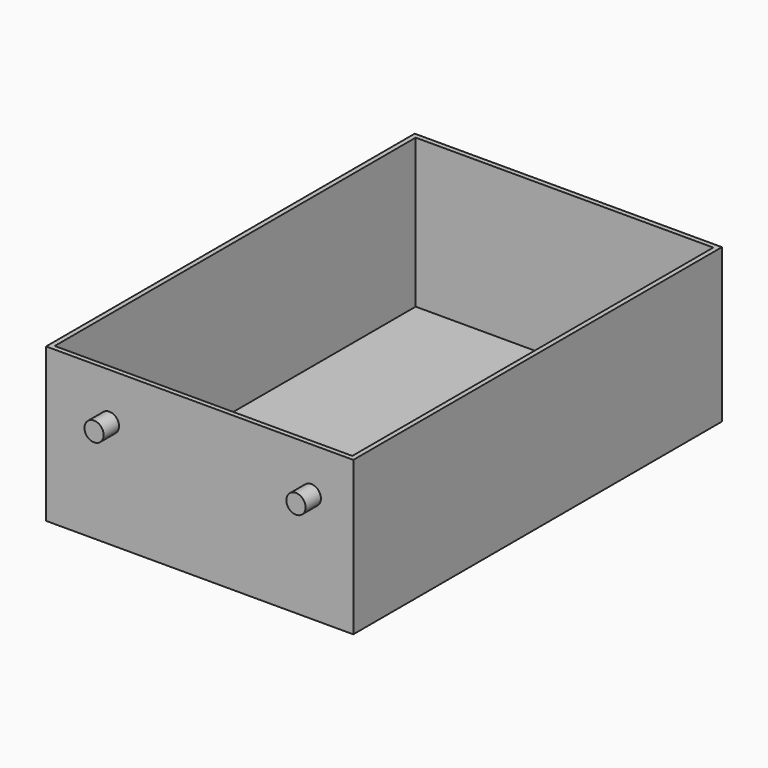
from build123d import *

# Parameters (mm, degrees)
F1_W      = 160
F1_H      = 80
F2_DEPTH  = 120
F5_T      = -2.5
F7_R      = 5
F9_DEPTH  = 10
F11_R     = 5
F12_DEPTH = 10


# Not quite as in the source:
# - the program builds the solid bodies; features that only make, move or delete a surface that nothing else refers to are left out


with BuildPart() as f2:
    # F1 (on face) → F2 (new body, symmetric)
    with BuildSketch(Plane.XZ):
        Rectangle(F1_W, F1_H)
    extrude(amount=F2_DEPTH, both=True)

    # F5
    f5_openings = [f2.faces().sort_by_distance(p)[0] for p in [
        (0, 0, 40),
    ]]
    offset(amount=F5_T, openings=f5_openings)

    # F11 (on face) → F12 (join)
    with BuildSketch(Plane(origin=(0, 120, 0), x_dir=(-1, 0, 0), z_dir=(0, 1, 0))):
        with Locations((-46.3621765375, 7.5514214113)):
            Circle(F11_R)
        with Locations((44.7815805674, 6.3221203163)):
            Circle(F11_R)
    extrude(amount=F12_DEPTH)


with BuildPart() as f9:
    # F7 (on face) → F9 (new body)
    with BuildSketch(Plane.XZ.offset(120)):
        with Locations((-47.0132157207, 15.8040374517)):
            Circle(F7_R)
    extrude(amount=F9_DEPTH)


with BuildPart() as f9b:
    # F7 (on face) → F9, piece 2 (new body)
    with BuildSketch(Plane.XZ.offset(120)):
        with Locations((58.1432282925, 16.818979755)):
            Circle(F7_R)
    extrude(amount=F9_DEPTH)


solid = Compound([f2.part, f9.part, f9b.part])
